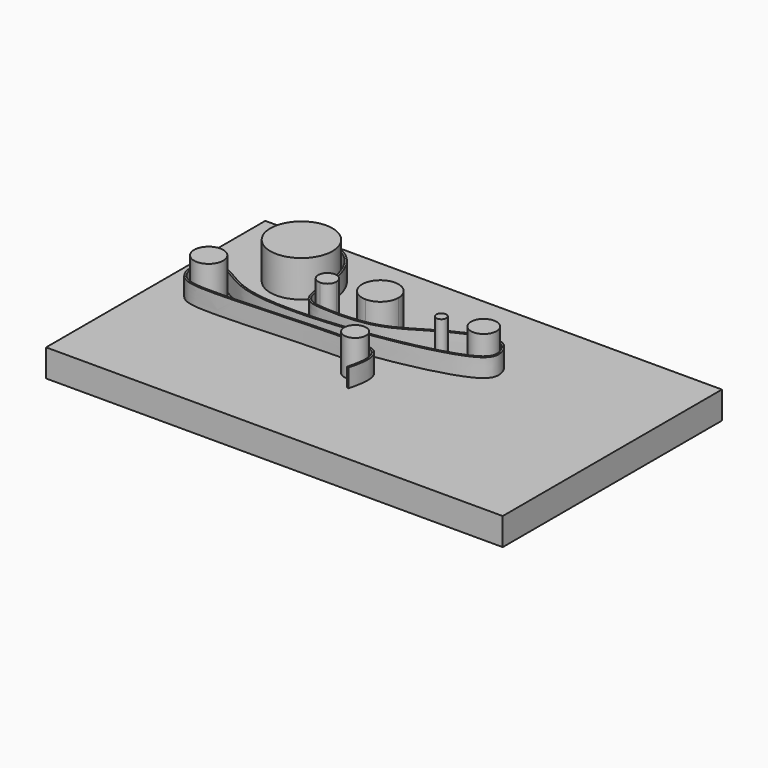
from build123d import *

# Parameters (mm, degrees)
F0_R     = 8
F1_DEPTH = 35
F0_R_2   = 17
F0_R_3   = 6
F0_R_4   = 7
F0_R_5   = 2.75
F0_W     = 250
F0_H     = 150
F2_DEPTH = 15
F3_DEPTH = 25


# Not quite as in the source:
# - ends of sketch curves that miss each other by under 0.0002 mm in the source are joined
# - the dataset's text gives a spline's control points without its knots; the knots are read off the source's solid


with BuildPart() as f1:
    # F0 (on Top) → F1 (new body)
    with BuildSketch(Plane.XY):
        with Locations((-88, 42)):
            Circle(F0_R)
    extrude(amount=F1_DEPTH)


with BuildPart() as f1b:
    # F0 (on Top) → F1, piece 2 (new body)
    with BuildSketch(Plane.XY):
        with Locations((-66, 78)):
            Circle(F0_R_2)
    extrude(amount=F1_DEPTH)


with BuildPart() as f1c:
    # F0 (on Top) → F1, piece 3 (new body)
    with BuildSketch(Plane.XY):
        with BuildLine():
            ThreePointArc((-35, 52), (-31.4644660941, 53.4644660941), (-30, 57))
            ThreePointArc((-30, 57), (-31.4644660941, 60.5355339059), (-35, 62))
            ThreePointArc((-35, 62), (-40, 57), (-35, 52))
        make_face()
    extrude(amount=F1_DEPTH)


with BuildPart() as f1d:
    # F0 (on Top) → F1, piece 4 (new body)
    with BuildSketch(Plane.XY):
        with BuildLine():
            ThreePointArc((0, 62), (-4.5227744249, 70.3666002653), (-14, 71.1651513899))
            ThreePointArc((-14, 71.1651513899), (-19.7890631293, 59.9569035631), (-10, 52))
            ThreePointArc((-10, 52), (-2.9289321881, 54.9289321881), (0, 62))
        make_face()
    extrude(amount=F1_DEPTH)


with BuildPart() as f1e:
    # F0 (on Top) → F1, piece 5 (new body)
    with BuildSketch(Plane.XY):
        with Locations((5, 26)):
            Circle(F0_R_3)
    extrude(amount=F1_DEPTH)


with BuildPart() as f1f:
    # F0 (on Top) → F1, piece 6 (new body)
    with BuildSketch(Plane.XY):
        with Locations((45, 64)):
            Circle(F0_R_4)
    extrude(amount=F1_DEPTH)


with BuildPart() as f1g:
    # F0 (on Top) → F1, piece 7 (new body)
    with BuildSketch(Plane.XY):
        with Locations((25, 60)):
            Circle(F0_R_5)
    extrude(amount=F1_DEPTH)


with BuildPart() as f2:
    # F0 (on Top) → F2 (new body)
    with BuildSketch(Plane.XY):
        with Locations((12, 37)):
            Rectangle(F0_W, F0_H)
        with Locations((5, 26)):
            Circle(F0_R_3, mode=Mode.SUBTRACT)
        with Locations((-88, 42)):
            Circle(F0_R, mode=Mode.SUBTRACT)
        with BuildLine():
            Line((-74.9913607382, 96.2543959587), (-75.2225406044, 97.2273081143))
            add(Edge.make_bspline(
                [(-75.2225406044, 97.2273081143), (-59.013935749, 101.078738153), (-40.7981644988, 83.8349148268), (-45.5017427759, 51.2859656792), (-29.429598885, 49.3489849199), (-1.804300878, 49.3534248671), (18.9989735418, 64.9177267653), (47.7812419345, 77.5858986316), (55.6233043112, 63.8665732673), (50.1596559628, 47.8330664354), (-67.8061882195, 29.8927833218), (-85.4649219142, 55.6140368465), (-99.6318258212, 45.5900481828), (-95.8566840113, 34.1790441633), (-81.3033786694, 29.6332256673), (4.2188295126, 37.4775677619), (13.1784604546, 30.2531227981), (14.2819178125, 23.0111152031), (11.6129393949, 13.069072922)],
                knots=[0, 0, 0, 0, 0.0733439387, 0.1394523519, 0.1830220548, 0.2482951719, 0.3152637608, 0.3814328622, 0.4227341159, 0.4664110955, 0.6006881165, 0.6648192323, 0.707078355, 0.7444100185, 0.7934656502, 0.9103644523, 0.9478554881, 1, 1, 1, 1], degree=3))
            Line((11.6129393949, 13.069072922), (10.6898449567, 13.4880220553))
            add(Edge.make_bspline(
                [(-74.9913607382, 96.2543959587), (-71.6298749078, 97.053140059), (-65.5437689688, 97.4969803696), (-58.2305813292, 95.4090888217), (-53.5108726624, 91.8838170684), (-50.5228162371, 88.2588098564), (-48.6773667774, 85.2096822283), (-47.2252953813, 81.9052980881), (-46.1759808526, 78.4240180546), (-45.4673421153, 74.8204726071), (-45.0063058383, 71.1823772796), (-44.7039270551, 67.5920644482), (-44.4670863312, 64.1313427999), (-44.2007881417, 60.8780038447), (-43.8720241959, 58.3995723979), (-43.4899688673, 56.5874426685), (-43.1272912257, 55.3201409625), (-42.6709439381, 54.1526567015), (-42.0938508009, 53.0911707018), (-41.3922756483, 52.1701587962), (-40.3101856463, 51.1301156883), (-38.7218576629, 50.1749961538), (-36.5495100981, 49.4700454599), (-34.1519328174, 49.0648883229), (-31.9782426094, 48.8797215842), (-30.1457141087, 48.7715285781), (-28.2433129983, 48.6754693041), (-25.7399162938, 48.5868739857), (-21.5280922616, 48.5405621049), (-15.9827300905, 48.7164571424), (-10.3485788091, 49.3519529468), (-5.9575165678, 50.2261537173), (-2.7631697745, 51.0923147938), (0.2828046916, 52.1777208932), (4.1943776898, 53.8685699577), (8.8893801075, 56.3671954287), (13.5688373308, 59.1851629613), (17.4516747072, 61.5224659907), (19.9670382752, 62.9958159089), (22.0518161572, 64.1692264089), (24.1883495835, 65.3340695966), (26.9323690909, 66.7529994114), (30.2764961357, 68.3323943269), (34.7122568159, 70.1885020653), (38.9760340039, 71.540953193), (42.7687074013, 72.1447653578), (44.8713333118, 72.1676359262), (46.3530660189, 71.9577640832), (47.3517902428, 71.6858123011), (48.2607707077, 71.296518943), (49.3643623324, 70.6377200138), (50.5507834681, 69.5762277829), (51.673454983, 68.0096072558), (52.3517006225, 66.5499355912), (52.7381609821, 65.3519362109), (52.9501752127, 64.4532647272), (53.0853674744, 63.5768415616), (53.1495047805, 62.4649027722), (52.9955094807, 61.1638498337), (52.3632305433, 59.6596541903), (51.1255235517, 58.1081555208), (49.4425780065, 56.763269524), (47.6425459104, 55.6659634721), (45.518130059, 54.555367278), (42.257410726, 53.1493335447), (37.5033113436, 51.4736049207), (32.0141634005, 49.8342608702), (23.8556683804, 47.7271874096), (12.3398880771, 45.2933866574), (-2.7761818921, 42.8541777446), (-18.3839283531, 41.0541398854), (-31.1290850704, 40.2173620285), (-40.7641331072, 40.0233949134), (-47.6079289577, 40.1346761293), (-53.966635019, 40.5212611317), (-58.7738176597, 41.0875375596), (-62.2720826939, 41.694469354), (-64.7051619471, 42.2282293707), (-66.9475141512, 42.8406766019), (-69.7074713557, 43.7422919713), (-72.758784475, 44.9948592117), (-75.8955967794, 46.5913083171), (-78.6195504235, 48.1766811664), (-81.0449381518, 49.6476092138), (-83.2924272509, 50.8988066686), (-85.130084797, 51.661341145), (-86.6417890212, 52.0239921786), (-87.8059929645, 52.1483179813), (-88.9962387178, 52.1000951461), (-90.5659003201, 51.8235028819), (-92.4743546409, 51.127052893), (-94.5748259458, 49.842245151), (-96.0804284554, 48.4734623159), (-97.0796520046, 47.2367438708), (-97.7095791561, 46.2469958326), (-98.2031982887, 45.1987394627), (-98.5331500741, 44.1132249549), (-98.7044994333, 43.0217670318), (-98.7417960728, 41.5727382343), (-98.4653061444, 39.8067669556), (-97.7285690188, 37.8348493569), (-96.6790151516, 36.0733498279), (-95.409783062, 34.5847104685), (-93.8435691718, 33.3683245233), (-91.9319487126, 32.4468308089), (-89.6250195574, 31.7887696564), (-86.8343119854, 31.3487457138), (-84.0186315115, 31.1325379675), (-81.4201552216, 31.0350737458), (-78.572016428, 30.9835746094), (-74.569261691, 30.9981788208), (-69.1643909353, 31.1206839903), (-63.2658775274, 31.3273173357), (-54.8893764716, 31.6873782791), (-43.7347862362, 32.2443228489), (-30.1421526706, 32.9185038775), (-19.3847662445, 33.3476224858), (-11.5689376833, 33.5289082389), (-6.2153952289, 33.5634091696), (-2.273299865, 33.4907398221), (0.5093374747, 33.3621444178), (2.3950807726, 33.2283213317), (4.0626799055, 33.0554241766), (5.4942133559, 32.8424192545), (6.7087184411, 32.5907463232), (8.0626963615, 32.2076053795), (9.3030705817, 31.6499307698), (10.1117927846, 31.01335336), (10.6285302272, 30.4246522791), (10.9735044032, 29.9287707455), (11.2990988402, 29.3621328199), (11.5936592598, 28.7545150331), (11.8519611539, 28.0920397091), (12.1437978529, 27.1156055107), (12.3971830535, 25.6829548599), (12.46919192, 23.5167059464), (12.1798523095, 19.943670112), (11.4560489575, 16.363063657), (10.6898449567, 13.4880220553)],
                knots=[0, 0, 0, 0, 0.015625, 0.03125, 0.046875, 0.0546875, 0.0625, 0.0703125, 0.078125, 0.0859375, 0.09375, 0.1015625, 0.109375, 0.1171875, 0.125, 0.12890625, 0.1328125, 0.13671875, 0.140625, 0.14453125, 0.1484375, 0.15625, 0.1640625, 0.171875, 0.1796875, 0.18359375, 0.1875, 0.1953125, 0.203125, 0.21875, 0.234375, 0.2421875, 0.25, 0.2578125, 0.265625, 0.28125, 0.296875, 0.3046875, 0.3125, 0.31640625, 0.3203125, 0.328125, 0.3359375, 0.34375, 0.359375, 0.3671875, 0.375, 0.37890625, 0.3828125, 0.38671875, 0.390625, 0.3984375, 0.40625, 0.4140625, 0.41796875, 0.421875, 0.42578125, 0.4296875, 0.4375, 0.4453125, 0.453125, 0.4609375, 0.46484375, 0.46875, 0.4765625, 0.484375, 0.4921875, 0.5, 0.515625, 0.53125, 0.546875, 0.5625, 0.5703125, 0.578125, 0.5859375, 0.59375, 0.59765625, 0.6015625, 0.60546875, 0.609375, 0.6171875, 0.625, 0.6328125, 0.640625, 0.6484375, 0.65625, 0.66015625, 0.6640625, 0.66796875, 0.671875, 0.6796875, 0.6875, 0.6953125, 0.69921875, 0.703125, 0.70703125, 0.7109375, 0.71484375, 0.71875, 0.7265625, 0.734375, 0.7421875, 0.75, 0.7578125, 0.765625, 0.7734375, 0.78125, 0.7890625, 0.79296875, 0.796875, 0.8046875, 0.8125, 0.8203125, 0.828125, 0.84375, 0.859375, 0.875, 0.8828125, 0.890625, 0.8984375, 0.90234375, 0.90625, 0.91015625, 0.9140625, 0.91796875, 0.921875, 0.9296875, 0.9375, 0.94140625, 0.9453125, 0.94921875, 0.953125, 0.95703125, 0.9609375, 0.96875, 0.9765625, 0.984375, 0.9997168928, 0.9997168928, 0.9997168928, 0.9997168928], degree=3))
        make_face(mode=Mode.SUBTRACT)
        with BuildLine():
            ThreePointArc((-35, 52), (-40, 57), (-35, 62))
            Line((-35, 62), (-14, 71.1651513899))
            ThreePointArc((-14, 71.1651513899), (-4.5227744249, 70.3666002653), (0, 62))
            ThreePointArc((0, 62), (-2.9289321881, 54.9289321881), (-10, 52))
            Line((-10, 52), (-35, 52))
        make_face(mode=Mode.SUBTRACT)
        with Locations((-66, 78)):
            Circle(F0_R_2, mode=Mode.SUBTRACT)
        with Locations((25, 60)):
            Circle(F0_R_5, mode=Mode.SUBTRACT)
        with Locations((45, 64)):
            Circle(F0_R_4, mode=Mode.SUBTRACT)
        with BuildLine():
            ThreePointArc((-35, 62), (-31.4644660941, 60.5355339059), (-30, 57))
            ThreePointArc((-30, 57), (-31.4644660941, 53.4644660941), (-35, 52))
            Line((-35, 52), (-10, 52))
            ThreePointArc((-10, 52), (-19.7890631293, 59.9569035631), (-14, 71.1651513899))
            Line((-14, 71.1651513899), (-35, 62))
        make_face()
    extrude(amount=F2_DEPTH)


with BuildPart() as f3:
    # F0 (on Top) → F3 (new body)
    with BuildSketch(Plane.XY):
        with BuildLine():
            add(Edge.make_bspline(
                [(-75.2225406044, 97.2273081143), (-59.013935749, 101.078738153), (-40.7981644988, 83.8349148268), (-45.5017427759, 51.2859656792), (-29.429598885, 49.3489849199), (-1.804300878, 49.3534248671), (18.9989735418, 64.9177267653), (47.7812419345, 77.5858986316), (55.6233043112, 63.8665732673), (50.1596559628, 47.8330664354), (-67.8061882195, 29.8927833218), (-85.4649219142, 55.6140368465), (-99.6318258212, 45.5900481828), (-95.8566840113, 34.1790441633), (-81.3033786694, 29.6332256673), (4.2188295126, 37.4775677619), (13.1784604546, 30.2531227981), (14.2819178125, 23.0111152031), (11.6129393949, 13.069072922)],
                knots=[0, 0, 0, 0, 0.0733439387, 0.1394523519, 0.1830220548, 0.2482951719, 0.3152637608, 0.3814328622, 0.4227341159, 0.4664110955, 0.6006881165, 0.6648192323, 0.707078355, 0.7444100185, 0.7934656502, 0.9103644523, 0.9478554881, 1, 1, 1, 1], degree=3))
            Line((-75.2225406044, 97.2273081143), (-74.9913607382, 96.2543959587))
            add(Edge.make_bspline(
                [(-74.9913607382, 96.2543959587), (-71.6298749078, 97.053140059), (-65.5437689688, 97.4969803696), (-58.2305813292, 95.4090888217), (-53.5108726624, 91.8838170684), (-50.5228162371, 88.2588098564), (-48.6773667774, 85.2096822283), (-47.2252953813, 81.9052980881), (-46.1759808526, 78.4240180546), (-45.4673421153, 74.8204726071), (-45.0063058383, 71.1823772796), (-44.7039270551, 67.5920644482), (-44.4670863312, 64.1313427999), (-44.2007881417, 60.8780038447), (-43.8720241959, 58.3995723979), (-43.4899688673, 56.5874426685), (-43.1272912257, 55.3201409625), (-42.6709439381, 54.1526567015), (-42.0938508009, 53.0911707018), (-41.3922756483, 52.1701587962), (-40.3101856463, 51.1301156883), (-38.7218576629, 50.1749961538), (-36.5495100981, 49.4700454599), (-34.1519328174, 49.0648883229), (-31.9782426094, 48.8797215842), (-30.1457141087, 48.7715285781), (-28.2433129983, 48.6754693041), (-25.7399162938, 48.5868739857), (-21.5280922616, 48.5405621049), (-15.9827300905, 48.7164571424), (-10.3485788091, 49.3519529468), (-5.9575165678, 50.2261537173), (-2.7631697745, 51.0923147938), (0.2828046916, 52.1777208932), (4.1943776898, 53.8685699577), (8.8893801075, 56.3671954287), (13.5688373308, 59.1851629613), (17.4516747072, 61.5224659907), (19.9670382752, 62.9958159089), (22.0518161572, 64.1692264089), (24.1883495835, 65.3340695966), (26.9323690909, 66.7529994114), (30.2764961357, 68.3323943269), (34.7122568159, 70.1885020653), (38.9760340039, 71.540953193), (42.7687074013, 72.1447653578), (44.8713333118, 72.1676359262), (46.3530660189, 71.9577640832), (47.3517902428, 71.6858123011), (48.2607707077, 71.296518943), (49.3643623324, 70.6377200138), (50.5507834681, 69.5762277829), (51.673454983, 68.0096072558), (52.3517006225, 66.5499355912), (52.7381609821, 65.3519362109), (52.9501752127, 64.4532647272), (53.0853674744, 63.5768415616), (53.1495047805, 62.4649027722), (52.9955094807, 61.1638498337), (52.3632305433, 59.6596541903), (51.1255235517, 58.1081555208), (49.4425780065, 56.763269524), (47.6425459104, 55.6659634721), (45.518130059, 54.555367278), (42.257410726, 53.1493335447), (37.5033113436, 51.4736049207), (32.0141634005, 49.8342608702), (23.8556683804, 47.7271874096), (12.3398880771, 45.2933866574), (-2.7761818921, 42.8541777446), (-18.3839283531, 41.0541398854), (-31.1290850704, 40.2173620285), (-40.7641331072, 40.0233949134), (-47.6079289577, 40.1346761293), (-53.966635019, 40.5212611317), (-58.7738176597, 41.0875375596), (-62.2720826939, 41.694469354), (-64.7051619471, 42.2282293707), (-66.9475141512, 42.8406766019), (-69.7074713557, 43.7422919713), (-72.758784475, 44.9948592117), (-75.8955967794, 46.5913083171), (-78.6195504235, 48.1766811664), (-81.0449381518, 49.6476092138), (-83.2924272509, 50.8988066686), (-85.130084797, 51.661341145), (-86.6417890212, 52.0239921786), (-87.8059929645, 52.1483179813), (-88.9962387178, 52.1000951461), (-90.5659003201, 51.8235028819), (-92.4743546409, 51.127052893), (-94.5748259458, 49.842245151), (-96.0804284554, 48.4734623159), (-97.0796520046, 47.2367438708), (-97.7095791561, 46.2469958326), (-98.2031982887, 45.1987394627), (-98.5331500741, 44.1132249549), (-98.7044994333, 43.0217670318), (-98.7417960728, 41.5727382343), (-98.4653061444, 39.8067669556), (-97.7285690188, 37.8348493569), (-96.6790151516, 36.0733498279), (-95.409783062, 34.5847104685), (-93.8435691718, 33.3683245233), (-91.9319487126, 32.4468308089), (-89.6250195574, 31.7887696564), (-86.8343119854, 31.3487457138), (-84.0186315115, 31.1325379675), (-81.4201552216, 31.0350737458), (-78.572016428, 30.9835746094), (-74.569261691, 30.9981788208), (-69.1643909353, 31.1206839903), (-63.2658775274, 31.3273173357), (-54.8893764716, 31.6873782791), (-43.7347862362, 32.2443228489), (-30.1421526706, 32.9185038775), (-19.3847662445, 33.3476224858), (-11.5689376833, 33.5289082389), (-6.2153952289, 33.5634091696), (-2.273299865, 33.4907398221), (0.5093374747, 33.3621444178), (2.3950807726, 33.2283213317), (4.0626799055, 33.0554241766), (5.4942133559, 32.8424192545), (6.7087184411, 32.5907463232), (8.0626963615, 32.2076053795), (9.3030705817, 31.6499307698), (10.1117927846, 31.01335336), (10.6285302272, 30.4246522791), (10.9735044032, 29.9287707455), (11.2990988402, 29.3621328199), (11.5936592598, 28.7545150331), (11.8519611539, 28.0920397091), (12.1437978529, 27.1156055107), (12.3971830535, 25.6829548599), (12.46919192, 23.5167059464), (12.1798523095, 19.943670112), (11.4560489575, 16.363063657), (10.6898444478, 13.4880221909)],
                knots=[0, 0, 0, 0, 0.015625, 0.03125, 0.046875, 0.0546875, 0.0625, 0.0703125, 0.078125, 0.0859375, 0.09375, 0.1015625, 0.109375, 0.1171875, 0.125, 0.12890625, 0.1328125, 0.13671875, 0.140625, 0.14453125, 0.1484375, 0.15625, 0.1640625, 0.171875, 0.1796875, 0.18359375, 0.1875, 0.1953125, 0.203125, 0.21875, 0.234375, 0.2421875, 0.25, 0.2578125, 0.265625, 0.28125, 0.296875, 0.3046875, 0.3125, 0.31640625, 0.3203125, 0.328125, 0.3359375, 0.34375, 0.359375, 0.3671875, 0.375, 0.37890625, 0.3828125, 0.38671875, 0.390625, 0.3984375, 0.40625, 0.4140625, 0.41796875, 0.421875, 0.42578125, 0.4296875, 0.4375, 0.4453125, 0.453125, 0.4609375, 0.46484375, 0.46875, 0.4765625, 0.484375, 0.4921875, 0.5, 0.515625, 0.53125, 0.546875, 0.5625, 0.5703125, 0.578125, 0.5859375, 0.59375, 0.59765625, 0.6015625, 0.60546875, 0.609375, 0.6171875, 0.625, 0.6328125, 0.640625, 0.6484375, 0.65625, 0.66015625, 0.6640625, 0.66796875, 0.671875, 0.6796875, 0.6875, 0.6953125, 0.69921875, 0.703125, 0.70703125, 0.7109375, 0.71484375, 0.71875, 0.7265625, 0.734375, 0.7421875, 0.75, 0.7578125, 0.765625, 0.7734375, 0.78125, 0.7890625, 0.79296875, 0.796875, 0.8046875, 0.8125, 0.8203125, 0.828125, 0.84375, 0.859375, 0.875, 0.8828125, 0.890625, 0.8984375, 0.90234375, 0.90625, 0.91015625, 0.9140625, 0.91796875, 0.921875, 0.9296875, 0.9375, 0.94140625, 0.9453125, 0.94921875, 0.953125, 0.95703125, 0.9609375, 0.96875, 0.9765625, 0.984375, 0.9997168928, 0.9997168928, 0.9997168928, 0.9997168928], degree=3))
            Line((10.6898444478, 13.4880221909), (11.6129393949, 13.069072922))
        make_face()
    extrude(amount=F3_DEPTH)


solid = Compound([f1.part, f1b.part, f1c.part, f1d.part, f1e.part, f1f.part, f1g.part, f2.part, f3.part])
